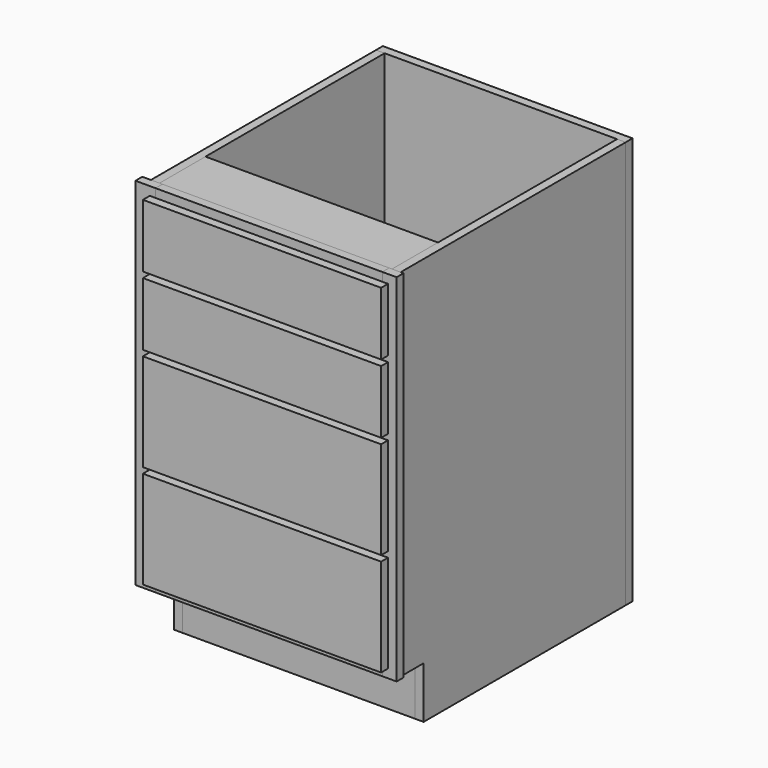
from build123d import *

# Parameters (mm, degrees)
F0_W      = 514.35
F0_H      = 19.05
F1_DEPTH  = 127
F2_W      = 19.05
F2_H      = 127
F3_DEPTH  = 19.05
F5_W      = 514.35
F5_H      = 603.25
F5_H_2    = 19.05
F6_DEPTH  = 19.05
F7_W      = 514.35
F7_H      = 127
F8_DEPTH  = 19.05
F9_W      = 501.65
F9_H      = 31.75
F10_DEPTH = 19.05
F11_DEPTH = 19.05
F9_W_2    = 19.05
F9_W_3    = 6.35
F9_H_2    = 723.9
F12_DEPTH = 19.05
F9_W_4    = 31.75
F13_DEPTH = 19.05
F9_H_3    = 38.1
F14_DEPTH = 19.05
F15_W     = 533.4
F15_H     = 901.7
F15_W_2   = 19.05
F16_DEPTH = 19.05
F17_W     = 527.05
F17_H     = 139.7
F18_DEPTH = 19.05
F17_H_2   = 215.9


with BuildPart() as f1:
    # F0 (on Top) → F1 (new body)
    with BuildSketch(Plane.XY):
        with Locations((0, 269.875)):
            Rectangle(F0_W, F0_H)
    extrude(amount=F1_DEPTH)


with BuildPart() as f1b:
    # F0 (on Top) → F1, piece 2 (new body)
    with BuildSketch(Plane.XY):
        with Locations((0, -269.875)):
            Rectangle(F0_W, F0_H)
    extrude(amount=F1_DEPTH)


with BuildPart() as f3:
    # F2 (on face) → F3 (new body)
    with BuildSketch(Plane(origin=(-257.175, 0, 0), x_dir=(0, -1, 0), z_dir=(-1, 0, 0))):
        Polygon((-260.35, 127), (-260.35, 0), (279.4, 0), (279.4, 114.3), (342.9, 114.3), (342.9, 901.7), (-279.4, 901.7), (-279.4, 127), align=None)
        with Locations((-269.875, 63.5)):
            Rectangle(F2_W, F2_H)
    extrude(amount=F3_DEPTH)


with BuildPart() as f4_1:
    # F4: instance of F3
    add(f3.part.mirror(Plane.YZ))


with BuildPart() as f6:
    # F5 (on face) → F6 (new body)
    with BuildSketch(Plane.XY.offset(127)):
        with Locations((0, -41.275)):
            Rectangle(F5_W, F5_H)
        with Locations((0, 269.875)):
            Rectangle(F5_W, F5_H_2)
    extrude(amount=F6_DEPTH)


with BuildPart() as f8:
    # F7 (on face) → F8 (new body)
    with BuildSketch(Plane.XY.offset(901.7)):
        with Locations((0, -279.4)):
            Rectangle(F7_W, F7_H)
    extrude(amount=-F8_DEPTH)


with BuildPart() as f10:
    # F9 (on face) → F10 (new body)
    with BuildSketch(Plane.XZ.offset(342.9)):
        with Locations((0, 885.825)):
            Rectangle(F9_W, F9_H)
    extrude(amount=F10_DEPTH)


with BuildPart() as f11:
    # F9 (on face) → F11 (new body)
    with BuildSketch(Plane.XZ.offset(342.9)):
        with Locations((0, 130.175)):
            Rectangle(F9_W, F9_H)
    extrude(amount=F11_DEPTH)


with BuildPart() as f11b:
    # F9 (on face) → F11, piece 2 (new body)
    with BuildSketch(Plane.XZ.offset(342.9)):
        with Locations((-266.7, 130.175)):
            Rectangle(F9_W_2, F9_H)
        with Locations((-279.4, 130.175)):
            Rectangle(F9_W_3, F9_H)
    extrude(amount=F11_DEPTH)

    # F9 (on face) → F12 (join)
    with BuildSketch(Plane.XZ.offset(342.9)):
        Polygon((-250.825, 869.95), (-257.175, 869.95), (-257.175, 146.05), (-250.825, 146.05), (-250.825, 336.55), (-250.825, 374.65), (-250.825, 565.15), (-250.825, 603.25), (-250.825, 717.55), (-250.825, 755.65), align=None)
        with Locations((-266.7, 508)):
            Rectangle(F9_W_2, F9_H_2)
        with Locations((-279.4, 508)):
            Rectangle(F9_W_3, F9_H_2)
        with Locations((-266.7, 885.825)):
            Rectangle(F9_W_2, F9_H)
        with Locations((-254, 885.825)):
            Rectangle(F9_W_3, F9_H)
        with Locations((-279.4, 885.825)):
            Rectangle(F9_W_3, F9_H)
        with Locations((-254, 130.175)):
            Rectangle(F9_W_3, F9_H)
        with Locations((-266.7, 130.175)):
            Rectangle(F9_W_2, F9_H)
        with Locations((-279.4, 130.175)):
            Rectangle(F9_W_3, F9_H)
        Polygon((-282.575, 869.95), (-282.575, 901.7), (-295.275, 901.7), (-295.275, 114.3), (-282.575, 114.3), (-282.575, 146.05), align=None)
    extrude(amount=F12_DEPTH)


with BuildPart() as f13:
    # F9 (on face) → F13 (new body)
    with BuildSketch(Plane.XZ.offset(342.9)):
        Polygon((282.575, 869.95), (250.825, 869.95), (250.825, 755.65), (250.825, 717.55), (250.825, 603.25), (250.825, 565.15), (250.825, 374.65), (250.825, 336.55), (250.825, 146.05), (282.575, 146.05), align=None)
        with Locations((266.7, 130.175)):
            Rectangle(F9_W_4, F9_H)
        with Locations((266.7, 885.825)):
            Rectangle(F9_W_4, F9_H)
    extrude(amount=F13_DEPTH)


with BuildPart() as f14:
    # F9 (on face) → F14 (new body)
    with BuildSketch(Plane.XZ.offset(342.9)):
        with Locations((0, 736.6)):
            Rectangle(F9_W, F9_H_3)
    extrude(amount=F14_DEPTH)


with BuildPart() as f14b:
    # F9 (on face) → F14, piece 2 (new body)
    with BuildSketch(Plane.XZ.offset(342.9)):
        with Locations((0, 355.6)):
            Rectangle(F9_W, F9_H_3)
    extrude(amount=F14_DEPTH)


with BuildPart() as f14c:
    # F9 (on face) → F14, piece 3 (new body)
    with BuildSketch(Plane.XZ.offset(342.9)):
        with Locations((0, 584.2)):
            Rectangle(F9_W, F9_H_3)
    extrude(amount=F14_DEPTH)


with BuildPart() as f16:
    # F15 (on face) → F16 (new body)
    with BuildSketch(Plane(origin=(0, 279.4, 0), x_dir=(-1, 0, 0), z_dir=(0, 1, 0))):
        with Locations((9.525, 450.85)):
            Rectangle(F15_W, F15_H)
        with Locations((-266.7, 450.85)):
            Rectangle(F15_W_2, F15_H)
    extrude(amount=F16_DEPTH)


with BuildPart() as f18:
    # F17 (on face) → F18 (new body)
    with BuildSketch(Plane.XZ.offset(361.95)):
        with Locations((0, 812.8)):
            Rectangle(F17_W, F17_H)
    extrude(amount=F18_DEPTH)


with BuildPart() as f18b:
    # F17 (on face) → F18, piece 2 (new body)
    with BuildSketch(Plane.XZ.offset(361.95)):
        with Locations((0, 660.4)):
            Rectangle(F17_W, F17_H)
    extrude(amount=F18_DEPTH)


with BuildPart() as f18c:
    # F17 (on face) → F18, piece 3 (new body)
    with BuildSketch(Plane.XZ.offset(361.95)):
        with Locations((0, 469.9)):
            Rectangle(F17_W, F17_H_2)
    extrude(amount=F18_DEPTH)


with BuildPart() as f18d:
    # F17 (on face) → F18, piece 4 (new body)
    with BuildSketch(Plane.XZ.offset(361.95)):
        with Locations((0, 241.3)):
            Rectangle(F17_W, F17_H_2)
    extrude(amount=F18_DEPTH)


solid = Compound([f1.part, f1b.part, f3.part, f4_1.part, f6.part, f8.part, f10.part, f11.part, f11b.part, f13.part, f14.part, f14b.part, f14c.part, f16.part, f18.part, f18b.part, f18c.part, f18d.part])
